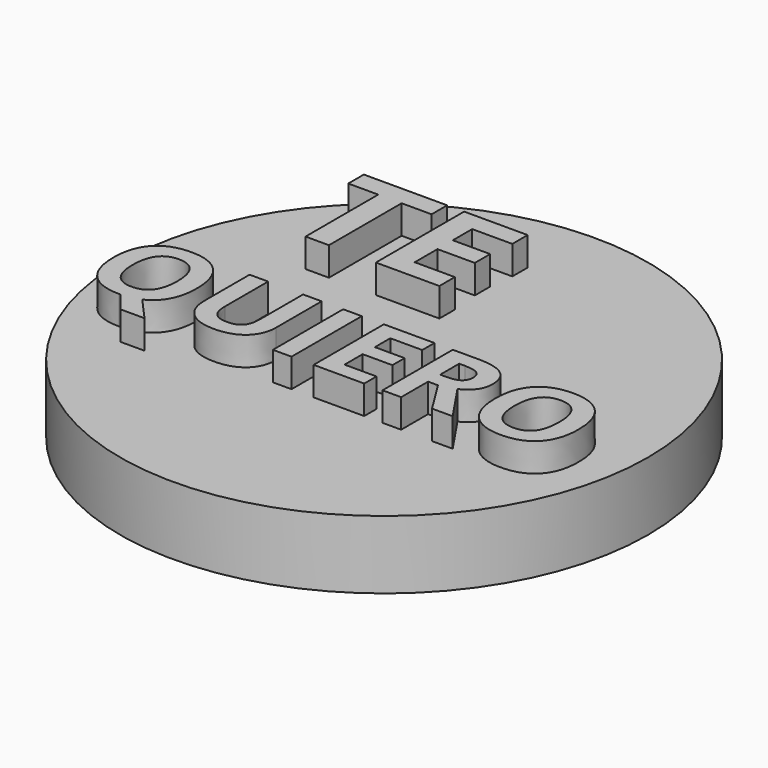
from build123d import *

# Parameters (mm, degrees)
F0_R         = 49.1638434115
F1_DEPTH     = 12.7
F2_TEXT_SIZE = 28.7861336621
F3_DEPTH     = 5.334
F4_TEXT_SIZE = 22.9126903125
F5_DEPTH     = 5.334


# Not quite as in the source:
# - Text() gives the source's letters only with a copy of the font that has no kerning and outlines rounded to 1/6400 em; it was checked with that copy


with BuildPart() as f1:
    # F0 (on Top) → F1 (new body)
    with BuildSketch(Plane.XY):
        Circle(F0_R)
    extrude(amount=F1_DEPTH)

    # F2 (on face) → F3 (join)
    with BuildSketch(Plane.XY.offset(12.7)):
        with Locations((-32.9556252097, 15.2095942758)):
            Text('TE', F2_TEXT_SIZE, font='Open Sans', font_style=FontStyle.BOLD, text_align=(TextAlign.LEFT, TextAlign.BOTTOM))
    extrude(amount=F3_DEPTH)

    # F4 (on face) → F5 (join)
    with BuildSketch(Plane.XY.offset(12.7)):
        with Locations((-45.8361469209, -15.6116015278)):
            Text('QUIERO', F4_TEXT_SIZE, font='Open Sans', font_style=FontStyle.BOLD, text_align=(TextAlign.LEFT, TextAlign.BOTTOM))
    extrude(amount=F5_DEPTH)


solid = f1.part
